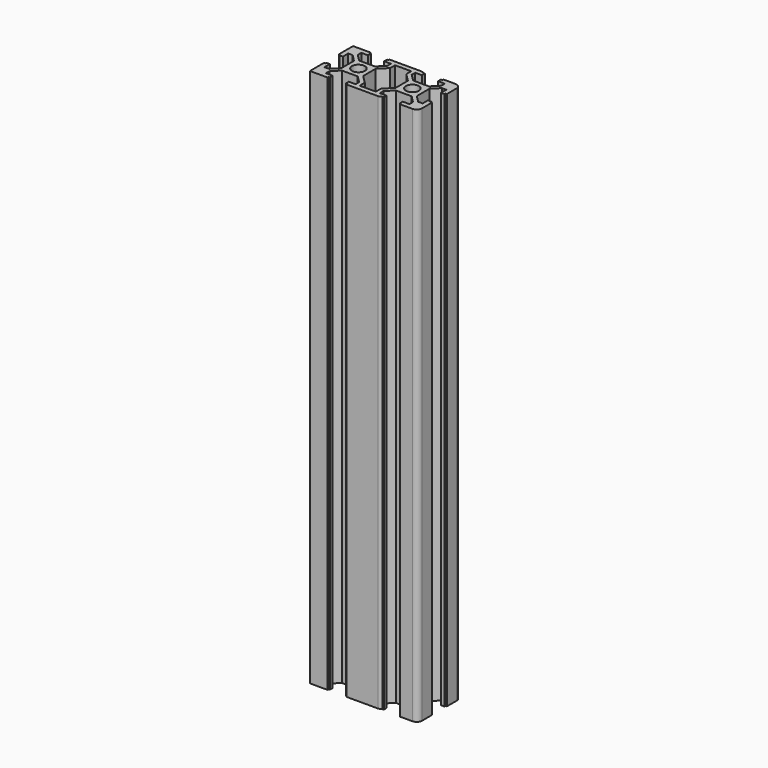
from build123d import *

# Parameters (mm, degrees)
F0_R        = 2.4
F1_DEPTH    = 200
F2_T1_DEPTH = 210
F2_T3_DEPTH = 206.6143782777
F3_R        = 1.5
F4_DEPTH    = 25


# Not quite as in the source:
# - a fillet or chamfer that OpenCascade refuses, or shapes differently, is made with other operations: its cross-section is extruded or revolved along the edge and cut away or added


with BuildPart() as f1:
    # F0 (on Top) → F1 (new body)
    with BuildSketch(Plane.XY):
        Polygon((10, 3.5), (10, 10), (3.5, 10), (3.5, 9.5), (3, 9.5), (3, 8.2), (5.5, 8.2), (5.5, 6.5606601718), (2.9393398282, 4), (0, 4), (-2.9393398282, 4), (-5.5, 6.5606601718), (-5.5, 8.2), (-3, 8.2), (-3, 9.5), (-3.5, 9.5), (-3.5, 10), (-10, 10), (-16.5, 10), (-16.5, 9.5), (-17, 9.5), (-17, 8.2), (-14.5, 8.2), (-14.5, 6.5606601718), (-17.0606601718, 4), (-20, 4), (-22.9393398282, 4), (-25.5, 6.5606601718), (-25.5, 8.2), (-23, 8.2), (-23, 9.5), (-23.5, 9.5), (-23.5, 10), (-30, 10), (-30, 3.5), (-29.5, 3.5), (-29.5, 3), (-28.2, 3), (-28.2, 5.5), (-26.5606601718, 5.5), (-24, 2.9393398282), (-24, -2.9393398282), (-26.5606601718, -5.5), (-28.2, -5.5), (-28.2, -3), (-29.5, -3), (-29.5, -3.5), (-30, -3.5), (-30, -10), (-23.5, -10), (-23.5, -9.5), (-23, -9.5), (-23, -8.2), (-25.5, -8.2), (-25.5, -6.5606601718), (-22.9393398282, -4), (-20, -4), (-17.0606601718, -4), (-14.5, -6.5606601718), (-14.5, -8.2), (-17, -8.2), (-17, -9.5), (-16.5, -9.5), (-16.5, -10), (-10, -10), (-3.5, -10), (-3.5, -9.5), (-3, -9.5), (-3, -8.2), (-5.5, -8.2), (-5.5, -6.5606601718), (-2.9393398282, -4), (0, -4), (2.9393398282, -4), (5.5, -6.5606601718), (5.5, -8.2), (3, -8.2), (3, -9.5), (3.5, -9.5), (3.5, -10), (10, -10), (10, -3.5), (9.5, -3.5), (9.5, -3), (8.2, -3), (8.2, -5.5), (6.5606601718, -5.5), (4, -2.9393398282), (4, 2.9393398282), (6.5606601718, 5.5), (8.2, 5.5), (8.2, 3), (9.5, 3), (9.5, 3.5), align=None)
        with Locations((-20, 0)):
            Circle(F0_R, mode=Mode.SUBTRACT)
        Polygon((-7, 5.9393398282), (-4, 2.9393398282), (-4, -2.797918472), (-7, -5.797918472), (-7, -8.2), (-13, -8.2), (-13, -5.797918472), (-16, -2.797918472), (-16, 2.9393398282), (-13, 5.9393398282), (-13, 8.2), (-7, 8.2), align=None, mode=Mode.SUBTRACT)
        Circle(F0_R, mode=Mode.SUBTRACT)
    extrude(amount=F1_DEPTH)

    # F2: fillet of radius 2 on 4 edges, made by hand

    # F2_s2 → F2_t1 (cut)
    with BuildSketch(Plane.XY.offset(-5)):
        with BuildLine():
            ThreePointArc((8, 10), (9.4142135624, 9.4142135624), (10, 8))
            Line((10, 8), (10, 10))
            Line((10, 10), (8, 10))
        make_face()
        with BuildLine():
            ThreePointArc((10, -8), (9.4142135624, -9.4142135624), (8, -10))
            Line((8, -10), (10, -10))
            Line((10, -10), (10, -8))
        make_face()
    extrude(amount=F2_T1_DEPTH, mode=Mode.SUBTRACT)

    # F2_s4 → F2_t3 (cut)
    with BuildSketch(Plane.XY.offset(-3.3071891388)):
        with BuildLine():
            ThreePointArc((-3.5, -9.5), (-4.1157688743, -9.8708286934), (-4.8228756555, -10))
            Line((-4.8228756555, -10), (-3.5, -10))
            Line((-3.5, -10), (-3.5, -9.5))
        make_face()
        with BuildLine():
            ThreePointArc((-4.8228756555, 10), (-4.1157688743, 9.8708286934), (-3.5, 9.5))
            Line((-3.5, 9.5), (-3.5, 10))
            Line((-3.5, 10), (-4.8228756555, 10))
        make_face()
    extrude(amount=F2_T3_DEPTH, mode=Mode.SUBTRACT)

    # F3 (on face) → F4 (cut)
    with BuildSketch(Plane.YZ.offset(4)):
        with Locations((0, 190.370157361)):
            Circle(F3_R)
    extrude(amount=-F4_DEPTH, mode=Mode.SUBTRACT)


solid = f1.part
